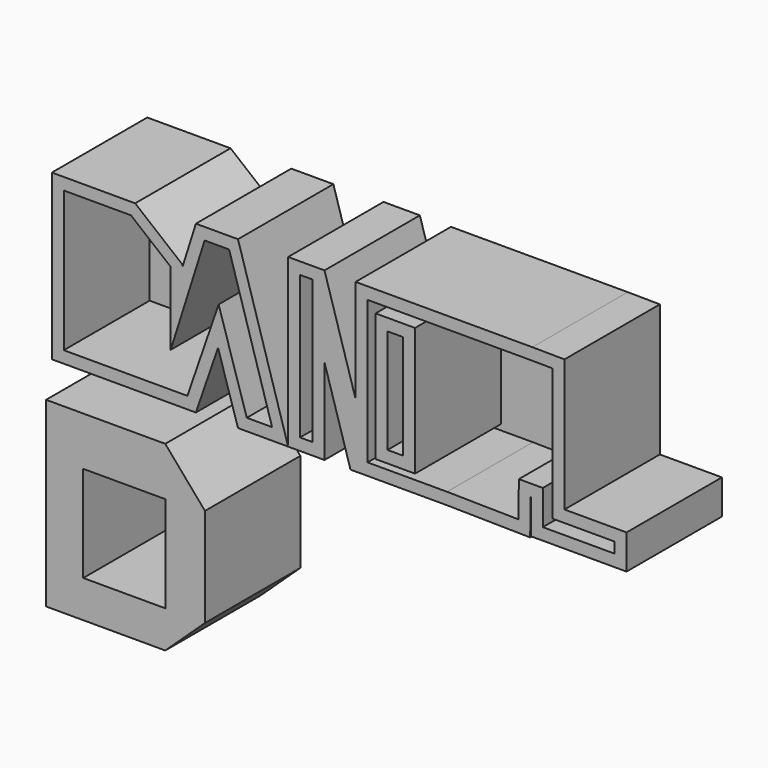
from build123d import *

# Parameters (mm, degrees)
F1_DEPTH    = 25.4
F3_DEPTH    = 25.4
F4_T        = -2.54
F5_T        = 2.54
F5_T3_DEPTH = 30.48
F6_W        = 17.4741521478
F6_H        = 20.4775221646
F7_DEPTH    = 25.4


# Not quite as in the source:
# - a shell that OpenCascade refuses in one call is made with other operations: the cavity is built on its own and cut out


with BuildPart() as f1:
    # F0 (on Front) → F1 (new body)
    with BuildSketch(Plane.XZ):
        Polygon((-7.751853343, 35.5700217187), (-7.751853343, 0), (0, 0), (0, 18.349380202), (5.5311000617, 0), (13.4272025898, 0), (13.4272025898, 5.9511377476), (13.4272025898, 6.2622595578), (13.4272025898, 28.5074785352), (13.4272025898, 35.5700217187), (6.6250464879, 35.5700217187), (6.6250464879, 13.591483), (0, 35.5700217187), align=None)
        Polygon((13.4272025898, 5.9511377476), (13.4272025898, 0), (26.0876882821, 0), (43.8216403127, -0.2713031718), (43.9208918573, 7.3511856608), (44.1983910351, 28.6630392075), (44.2883260548, 35.5700217187), (26.0876882821, 35.5700217187), (13.4272025898, 35.5700217187), (13.4272025898, 28.5074785352), (16.7540293187, 28.5074785352), (16.7540293187, 6.2622595578), (13.4272025898, 6.2622595578), align=None)
        Polygon((51.1330030859, 35.5077236891), (44.2883260548, 35.5700217187), (44.2883260548, 28.6630392075), (44.1983910351, 28.6630392075), (43.9208918573, 7.3511856608), (43.977200985, 7.3511856608), (43.977200985, 0), (64.355686307, 0), (64.355686307, 7.3511856608), (51.1330030859, 7.3511856608), align=None)
        Polygon((44.2883260548, 28.6630392075), (44.2883260548, 35.5700217187), (44.1983910351, 28.6630392075), align=None)
    extrude(amount=F1_DEPTH)

    # F5: shell of thickness 2.54, made by hand


with BuildPart() as f1b:
    # F0 (on Front) → F1, piece 2 (new body)
    with BuildSketch(Plane.XZ):
        Polygon((-27.4027399719, 35.4263968766), (-38.5948903859, 0), (-27.4027399719, 0), (-22.6853881031, 13.6895719916), (-18.4305217117, 0), (-7.751853343, 0), (-18.4305217117, 35.4263968766), align=None)
    extrude(amount=F1_DEPTH)

    # F2 (on Front) → F3 (join)
    with BuildSketch(Plane.XZ):
        Polygon((-58.0855421722, 35.0350737572), (-58.0855421722, 0), (-38.4715683758, 0), (-30.226835981, 11.0594791437), (-30.226835981, 26.7903394997), (-40.3383001685, 35.0350737572), align=None)
    extrude(amount=F3_DEPTH)

    # F4
    f4_openings = [f1b.faces().sort_by_distance(p)[0] for p in [
        (-36.054344, -25.4, 16.831568),
    ]]
    offset(amount=F4_T, openings=f4_openings, kind=Kind.INTERSECTION)


with BuildPart() as f5_core1:
    # F5_t2: copy of F1
    add(f1.part)

    # the walls: a layer under each face that stays
    f5_faces = [f5_core1.faces().sort_by_distance(p)[0] for p in [
        (47.7106645703, -12.7, 35.5388727039),
        (25.4566862714, -12.7, 35.5700217187),
        (6.6250464879, -12.7, 24.5807523594),
        (3.3125232439, -12.7, 24.5807523594),
        (-3.8759266715, -12.7, 35.5700217187),
        (-7.751853343, -12.7, 17.7850108594),
        (-3.8759266715, -12.7, 0),
        (0, -12.7, 9.174690101),
        (2.7655500308, -12.7, 9.174690101),
        (15.8093941719, -12.7, 0),
        (34.9546642974, -12.7, -0.1356515859),
        (43.871266085, -12.7, 3.5399412445),
        (43.9490464211, -12.7, 7.3511856608),
        (43.977200985, -12.7, 3.6755928304),
        (54.166443646, -12.7, 0),
        (64.355686307, -12.7, 3.6755928304),
        (57.7443446964, -12.7, 7.3511856608),
        (51.1330030859, -12.7, 21.4294546749),
        (13.4272025898, -12.7, 17.3848690465),
        (15.0906159543, -12.7, 28.5074785352),
        (16.7540293187, -12.7, 17.3848690465),
        (15.0906159543, -12.7, 6.2622595578),
        (28.301916482, 0, 17.6493592735),
    ]]
    thicken(f5_faces, amount=-F5_T, mode=Mode.SUBTRACT)

    # F5_s4 → F5_t3 (cut)
    with BuildSketch(Plane.XZ.offset(-2.54)):
        Polygon((6.6239656661, 13.5988135914), (9.1650464879, 13.591483), (9.1650464879, -3.6358737387), (4.1931286643, 12.8584238625), align=None)
        Polygon((0.0010808218, 18.3420496106), (-2.54, 18.349380202), (-2.54, 35.5767369407), (2.4319178236, 19.0824393395), align=None)
        Polygon((26.0872997453, -0.0507970282), (26.0876882821, 2.54), (26.1071162624, 2.54), (26.1265419696, 2.5397028155), align=None)
        Polygon((43.9462897044, 7.3254549584), (41.3811071501, 7.3842559035), (41.4137495922, 9.8911856608), (43.9208918573, 9.8911856608), align=None)
        Polygon((43.951800985, 7.3257856608), (43.977200985, 9.8911856608), (46.517200985, 9.8911856608), (46.517200985, 7.3511856608), align=None)
        Polygon((51.1584030859, 7.3765856608), (51.1330030859, 4.8111856608), (48.5930030859, 4.8111856608), (48.5930030859, 7.3511856608), align=None)
        Polygon((13.4526025898, 6.2876595578), (10.8872025898, 6.2622595578), (10.8872025898, 3.7222595578), (13.4272025898, 3.7222595578), align=None)
        Polygon((13.4526025898, 28.4820785352), (10.8872025898, 28.5074785352), (10.8872025898, 31.0474785352), (13.4272025898, 31.0474785352), align=None)
        Polygon((16.7286293187, 28.4820785352), (16.7540293187, 31.0474785352), (19.2940293187, 31.0474785352), (19.2940293187, 28.5074785352), align=None)
        Polygon((16.7286293187, 6.2876595578), (19.2940293187, 6.2622595578), (19.2940293187, 3.7222595578), (16.7540293187, 3.7222595578), align=None)
    extrude(amount=F5_T3_DEPTH, mode=Mode.SUBTRACT)


with BuildPart() as f1_1:
    add(f1.part)

    # what is left inside the walls is the cavity
    f5_cavity = [f5_core1.part.solids().sort_by_distance(p)[0] for p in [
        (35.490366, -2.5654, 12.548235),
        (-5.186453, -17.78, 17.785011),
    ]]
    add(f5_cavity, mode=Mode.SUBTRACT)


with BuildPart() as f7:
    # F6 (on Front) → F7 (new body)
    with BuildSketch(Plane.XZ):
        Polygon((-33.9281708002, -7.9899784178), (-59.3202970922, -7.9899784178), (-59.3202970922, -46.7607527971), (-33.9281708002, -46.7607527971), (-25.4641305655, -38.8427786529), (-25.4641305655, -17.8191885352), align=None)
        with Locations((-42.6652468741, -28.6040175706)):
            Rectangle(F6_W, F6_H, mode=Mode.SUBTRACT)
    extrude(amount=F7_DEPTH)


solid = Compound([f1b.part, f1_1.part, f7.part])
